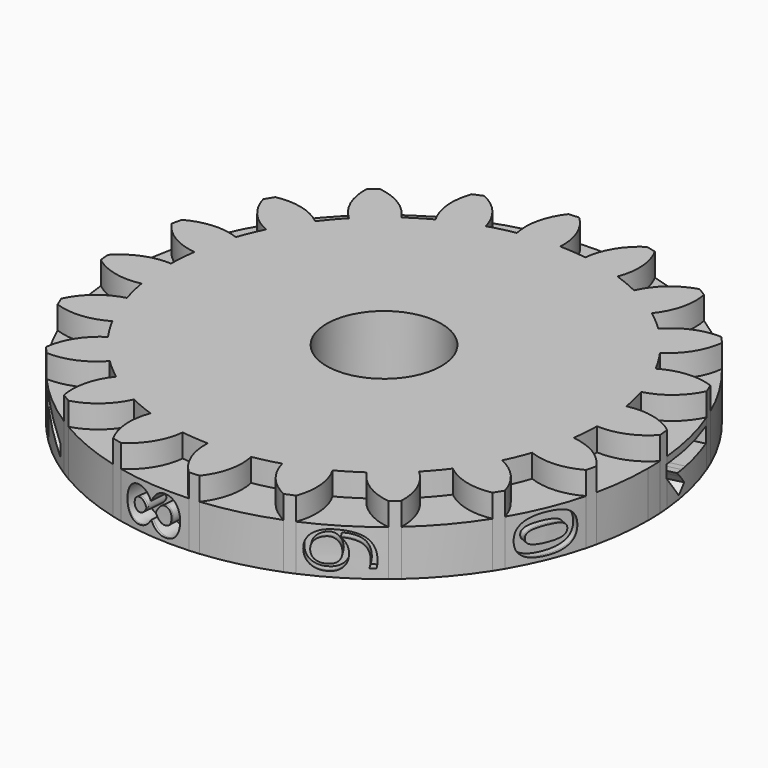
from build123d import *

# Parameters (mm, degrees)
F1_R          = 3.5
F1_R_2        = 2.5
F2_DEPTH      = 3
F3_DEPTH      = 2
F4_DEPTH      = 1
F8_TEXT_SIZE  = 3.422459893
F9_DEPTH      = 0.25
F11_TEXT_SIZE = 3.242330425
F12_DEPTH     = 0.25
F14_TEXT_SIZE = 3.3822665884
F15_DEPTH     = 0.25
F17_TEXT_SIZE = 3.3391304348
F18_DEPTH     = 0.25
F20_TEXT_SIZE = 4.3570347958
F21_DEPTH     = 0.9
F23_TEXT_SIZE = 3.3635036496
F24_DEPTH     = 0.25
F26_TEXT_SIZE = 3.4740651387
F27_DEPTH     = 0.25
F29_TEXT_SIZE = 3.3576216846
F30_DEPTH     = 0.9
F32_TEXT_SIZE = 3.3391304348
F33_DEPTH     = 0.25
F35_TEXT_SIZE = 3.3391304348
F36_DEPTH     = 0.25
F37_R         = 3.5
F37_R_2       = 2.5
F38_DEPTH     = 1


# Not quite as in the source:
# - Text() gives the source's letters only with a copy of the font that has no kerning and outlines rounded to 1/6400 em; it was checked with that copy


with BuildPart() as f2:
    # F1 (on Top) → F2 (new body)
    with BuildSketch(Plane.XY):
        with BuildLine():
            ThreePointArc((9.4078443957, -0.1531520845), (9.4087792756, -0.0765785786), (9.4090909091, 0))
            ThreePointArc((9.4090909091, 0), (9.3737668631, 0.8145468262), (9.2680599554, 1.6229776334))
            ThreePointArc((9.2680599554, 1.6229776334), (9.1491169783, 2.1965086508), (8.9947183137, 2.7615275108))
            ThreePointArc((8.9947183137, 2.7615275108), (8.6928665104, 3.6007032045), (8.3129211438, 4.4075314852))
            ThreePointArc((8.3129211438, 4.4075314852), (8.0225688191, 4.9162364953), (7.7011265332, 5.4058895526))
            ThreePointArc((7.7011265332, 5.4058895526), (7.1547288581, 6.1107157275), (6.5440556911, 6.7606454461))
            ThreePointArc((6.5440556911, 6.7606454461), (6.1107157275, 7.1547288581), (5.6536948308, 7.52108546))
            ThreePointArc((5.6536948308, 7.52108546), (4.9162364953, 8.0225688191), (4.1346124722, 8.4519803265))
            ThreePointArc((4.1346124722, 8.4519803265), (3.6007032045, 8.6928665104), (3.0528400867, 8.90006512))
            ThreePointArc((3.0528400867, 8.90006512), (2.1965086508, 9.1491169783), (1.320444577, 9.3159764842))
            ThreePointArc((1.320444577, 9.3159764842), (0.7382287643, 9.3800858219), (0.1531520845, 9.4078443957))
            ThreePointArc((0.1531520845, 9.4078443957), (-0.7382287643, 9.3800858219), (-1.6229776334, 9.2680599554))
            ThreePointArc((-1.6229776334, 9.2680599554), (-2.1965086508, 9.1491169783), (-2.7615275108, 8.9947183137))
            ThreePointArc((-2.7615275108, 8.9947183137), (-3.6007032045, 8.6928665104), (-4.4075314852, 8.3129211438))
            ThreePointArc((-4.4075314852, 8.3129211438), (-4.9162364953, 8.0225688191), (-5.4058895526, 7.7011265332))
            ThreePointArc((-5.4058895526, 7.7011265332), (-6.1107157275, 7.1547288581), (-6.7606454461, 6.5440556911))
            ThreePointArc((-6.7606454461, 6.5440556911), (-7.1547288581, 6.1107157275), (-7.52108546, 5.6536948308))
            ThreePointArc((-7.52108546, 5.6536948308), (-8.0225688191, 4.9162364953), (-8.4519803265, 4.1346124722))
            ThreePointArc((-8.4519803265, 4.1346124722), (-8.6928665104, 3.6007032045), (-8.90006512, 3.0528400867))
            ThreePointArc((-8.90006512, 3.0528400867), (-9.1491169783, 2.1965086508), (-9.3159764842, 1.320444577))
            ThreePointArc((-9.3159764842, 1.320444577), (-9.3800858219, 0.7382287643), (-9.4078443957, 0.1531520845))
            ThreePointArc((-9.4078443957, 0.1531520845), (-9.3800858219, -0.7382287643), (-9.2680599554, -1.6229776334))
            ThreePointArc((-9.2680599554, -1.6229776334), (-9.1491169783, -2.1965086508), (-8.9947183137, -2.7615275108))
            ThreePointArc((-8.9947183137, -2.7615275108), (-8.6928665104, -3.6007032045), (-8.3129211438, -4.4075314852))
            ThreePointArc((-8.3129211438, -4.4075314852), (-8.0225688191, -4.9162364953), (-7.7011265332, -5.4058895526))
            ThreePointArc((-7.7011265332, -5.4058895526), (-7.1547288581, -6.1107157275), (-6.5440556911, -6.7606454461))
            ThreePointArc((-6.5440556911, -6.7606454461), (-6.1107157275, -7.1547288581), (-5.6536948308, -7.52108546))
            ThreePointArc((-5.6536948308, -7.52108546), (-4.9162364953, -8.0225688191), (-4.1346124722, -8.4519803265))
            ThreePointArc((-4.1346124722, -8.4519803265), (-3.6007032045, -8.6928665104), (-3.0528400867, -8.90006512))
            ThreePointArc((-3.0528400867, -8.90006512), (-2.1965086508, -9.1491169783), (-1.320444577, -9.3159764842))
            ThreePointArc((-1.320444577, -9.3159764842), (-0.7382287643, -9.3800858219), (-0.1531520845, -9.4078443957))
            ThreePointArc((-0.1531520845, -9.4078443957), (0.7382287643, -9.3800858219), (1.6229776334, -9.2680599554))
            ThreePointArc((1.6229776334, -9.2680599554), (2.1965086508, -9.1491169783), (2.7615275108, -8.9947183137))
            ThreePointArc((2.7615275108, -8.9947183137), (3.6007032045, -8.6928665104), (4.4075314852, -8.3129211438))
            ThreePointArc((4.4075314852, -8.3129211438), (4.9162364953, -8.0225688191), (5.4058895526, -7.7011265332))
            ThreePointArc((5.4058895526, -7.7011265332), (6.1107157275, -7.1547288581), (6.7606454461, -6.5440556911))
            ThreePointArc((6.7606454461, -6.5440556911), (7.1547288581, -6.1107157275), (7.52108546, -5.6536948308))
            ThreePointArc((7.52108546, -5.6536948308), (8.0225688191, -4.9162364953), (8.4519803265, -4.1346124722))
            ThreePointArc((8.4519803265, -4.1346124722), (8.6928665104, -3.6007032045), (8.90006512, -3.0528400867))
            ThreePointArc((8.90006512, -3.0528400867), (9.1491169783, -2.1965086508), (9.3159764842, -1.320444577))
            ThreePointArc((9.3159764842, -1.320444577), (9.3800858219, -0.7382287643), (9.4078443957, -0.1531520845))
        make_face()
        Circle(F1_R, mode=Mode.SUBTRACT)
        Circle(F1_R)
        Circle(F1_R_2, mode=Mode.SUBTRACT)
        with BuildLine():
            ThreePointArc((-9.2680599554, -1.6229776334), (-9.3800858219, -0.7382287643), (-9.4078443957, 0.1531520845))
            ThreePointArc((-9.4078443957, 0.1531520845), (-10.5374998224, -0.0317997207), (-11.4797736507, -0.6817601701))
            Line((-11.4797736507, -0.6817601701), (-11.4450893749, -1.1224656787))
            ThreePointArc((-11.4450893749, -1.1224656787), (-10.4127402859, -1.6170199342), (-9.2680599554, -1.6229776334))
        make_face()
        with BuildLine():
            ThreePointArc((-9.3159764842, 1.320444577), (-9.1491169783, 2.1965086508), (-8.90006512, 3.0528400867))
            ThreePointArc((-8.90006512, 3.0528400867), (-10.0315845257, 3.2260231917), (-11.1285890147, 2.8990526973))
            Line((-11.1285890147, 2.8990526973), (-11.2317877999, 2.469198821))
            ThreePointArc((-11.2317877999, 2.469198821), (-10.4027911413, 1.679836361), (-9.3159764842, 1.320444577))
        make_face()
    extrude(amount=-F2_DEPTH)

    # F1 (on Top) → F3 (join)
    with BuildSketch(Plane.XY):
        with BuildLine():
            ThreePointArc((9.4078443957, -0.1531520845), (9.4087792756, -0.0765785786), (9.4090909091, 0))
            ThreePointArc((9.4090909091, 0), (9.3737668631, 0.8145468262), (9.2680599554, 1.6229776334))
            ThreePointArc((9.2680599554, 1.6229776334), (9.1491169783, 2.1965086508), (8.9947183137, 2.7615275108))
            ThreePointArc((8.9947183137, 2.7615275108), (8.6928665104, 3.6007032045), (8.3129211438, 4.4075314852))
            ThreePointArc((8.3129211438, 4.4075314852), (8.0225688191, 4.9162364953), (7.7011265332, 5.4058895526))
            ThreePointArc((7.7011265332, 5.4058895526), (7.1547288581, 6.1107157275), (6.5440556911, 6.7606454461))
            ThreePointArc((6.5440556911, 6.7606454461), (6.1107157275, 7.1547288581), (5.6536948308, 7.52108546))
            ThreePointArc((5.6536948308, 7.52108546), (4.9162364953, 8.0225688191), (4.1346124722, 8.4519803265))
            ThreePointArc((4.1346124722, 8.4519803265), (3.6007032045, 8.6928665104), (3.0528400867, 8.90006512))
            ThreePointArc((3.0528400867, 8.90006512), (2.1965086508, 9.1491169783), (1.320444577, 9.3159764842))
            ThreePointArc((1.320444577, 9.3159764842), (0.7382287643, 9.3800858219), (0.1531520845, 9.4078443957))
            ThreePointArc((0.1531520845, 9.4078443957), (-0.7382287643, 9.3800858219), (-1.6229776334, 9.2680599554))
            ThreePointArc((-1.6229776334, 9.2680599554), (-2.1965086508, 9.1491169783), (-2.7615275108, 8.9947183137))
            ThreePointArc((-2.7615275108, 8.9947183137), (-3.6007032045, 8.6928665104), (-4.4075314852, 8.3129211438))
            ThreePointArc((-4.4075314852, 8.3129211438), (-4.9162364953, 8.0225688191), (-5.4058895526, 7.7011265332))
            ThreePointArc((-5.4058895526, 7.7011265332), (-6.1107157275, 7.1547288581), (-6.7606454461, 6.5440556911))
            ThreePointArc((-6.7606454461, 6.5440556911), (-7.1547288581, 6.1107157275), (-7.52108546, 5.6536948308))
            ThreePointArc((-7.52108546, 5.6536948308), (-8.0225688191, 4.9162364953), (-8.4519803265, 4.1346124722))
            ThreePointArc((-8.4519803265, 4.1346124722), (-8.6928665104, 3.6007032045), (-8.90006512, 3.0528400867))
            ThreePointArc((-8.90006512, 3.0528400867), (-9.1491169783, 2.1965086508), (-9.3159764842, 1.320444577))
            ThreePointArc((-9.3159764842, 1.320444577), (-9.3800858219, 0.7382287643), (-9.4078443957, 0.1531520845))
            ThreePointArc((-9.4078443957, 0.1531520845), (-9.3800858219, -0.7382287643), (-9.2680599554, -1.6229776334))
            ThreePointArc((-9.2680599554, -1.6229776334), (-9.1491169783, -2.1965086508), (-8.9947183137, -2.7615275108))
            ThreePointArc((-8.9947183137, -2.7615275108), (-8.6928665104, -3.6007032045), (-8.3129211438, -4.4075314852))
            ThreePointArc((-8.3129211438, -4.4075314852), (-8.0225688191, -4.9162364953), (-7.7011265332, -5.4058895526))
            ThreePointArc((-7.7011265332, -5.4058895526), (-7.1547288581, -6.1107157275), (-6.5440556911, -6.7606454461))
            ThreePointArc((-6.5440556911, -6.7606454461), (-6.1107157275, -7.1547288581), (-5.6536948308, -7.52108546))
            ThreePointArc((-5.6536948308, -7.52108546), (-4.9162364953, -8.0225688191), (-4.1346124722, -8.4519803265))
            ThreePointArc((-4.1346124722, -8.4519803265), (-3.6007032045, -8.6928665104), (-3.0528400867, -8.90006512))
            ThreePointArc((-3.0528400867, -8.90006512), (-2.1965086508, -9.1491169783), (-1.320444577, -9.3159764842))
            ThreePointArc((-1.320444577, -9.3159764842), (-0.7382287643, -9.3800858219), (-0.1531520845, -9.4078443957))
            ThreePointArc((-0.1531520845, -9.4078443957), (0.7382287643, -9.3800858219), (1.6229776334, -9.2680599554))
            ThreePointArc((1.6229776334, -9.2680599554), (2.1965086508, -9.1491169783), (2.7615275108, -8.9947183137))
            ThreePointArc((2.7615275108, -8.9947183137), (3.6007032045, -8.6928665104), (4.4075314852, -8.3129211438))
            ThreePointArc((4.4075314852, -8.3129211438), (4.9162364953, -8.0225688191), (5.4058895526, -7.7011265332))
            ThreePointArc((5.4058895526, -7.7011265332), (6.1107157275, -7.1547288581), (6.7606454461, -6.5440556911))
            ThreePointArc((6.7606454461, -6.5440556911), (7.1547288581, -6.1107157275), (7.52108546, -5.6536948308))
            ThreePointArc((7.52108546, -5.6536948308), (8.0225688191, -4.9162364953), (8.4519803265, -4.1346124722))
            ThreePointArc((8.4519803265, -4.1346124722), (8.6928665104, -3.6007032045), (8.90006512, -3.0528400867))
            ThreePointArc((8.90006512, -3.0528400867), (9.1491169783, -2.1965086508), (9.3159764842, -1.320444577))
            ThreePointArc((9.3159764842, -1.320444577), (9.3800858219, -0.7382287643), (9.4078443957, -0.1531520845))
        make_face()
        Circle(F1_R, mode=Mode.SUBTRACT)
        Circle(F1_R)
        Circle(F1_R_2, mode=Mode.SUBTRACT)
        with BuildLine():
            ThreePointArc((4.195837602, -10.7072380574), (3.286509855, -10.0119312174), (2.7615275108, -8.9947183137))
            ThreePointArc((2.7615275108, -8.9947183137), (2.1965086508, -9.1491169783), (1.6229776334, -9.2680599554))
            ThreePointArc((1.6229776334, -9.2680599554), (1.6170199342, -10.4127402859), (1.1224656787, -11.4450893749))
            ThreePointArc((1.1224656787, -11.4450893749), (2.6846216843, -11.1822540846), (4.195837602, -10.7072380574))
        make_face()
        with BuildLine():
            ThreePointArc((7.2991972152, -8.8866034014), (6.2195135061, -8.5063250277), (5.4058895526, -7.7011265332))
            ThreePointArc((5.4058895526, -7.7011265332), (4.9162364953, -8.0225688191), (4.4075314852, -8.3129211438))
            ThreePointArc((4.4075314852, -8.3129211438), (4.7555910517, -9.4034178615), (4.604255417, -10.5380658593))
            ThreePointArc((4.604255417, -10.5380658593), (6.0087334942, -9.8053618901), (7.2991972152, -8.8866034014))
        make_face()
        with BuildLine():
            ThreePointArc((9.6880605486, -6.1960860878), (8.5437078414, -6.1680604771), (7.52108546, -5.6536948308))
            ThreePointArc((7.52108546, -5.6536948308), (7.1547288581, -6.1107157275), (6.7606454461, -6.5440556911))
            ThreePointArc((6.7606454461, -6.5440556911), (7.428651783, -7.4736233793), (7.6353485554, -8.5995030343))
            ThreePointArc((7.6353485554, -8.5995030343), (8.7446686044, -7.4686525558), (9.6880605486, -6.1960860878))
        make_face()
        with BuildLine():
            ThreePointArc((11.1285890147, -2.8990526973), (10.0315845257, -3.2260231917), (8.90006512, -3.0528400867))
            ThreePointArc((8.90006512, -3.0528400867), (8.6928665104, -3.6007032045), (8.4519803265, -4.1346124722))
            ThreePointArc((8.4519803265, -4.1346124722), (9.3745443193, -4.812258569), (9.9190405786, -5.8191609361))
            ThreePointArc((9.9190405786, -5.8191609361), (10.6246146239, -4.4008594722), (11.1285890147, -2.8990526973))
        make_face()
        with BuildLine():
            ThreePointArc((11.4797736507, 0.6817601701), (10.5374998224, 0.0317997207), (9.4078443957, -0.1531520845))
            ThreePointArc((9.4078443957, -0.1531520845), (9.3800858219, -0.7382287643), (9.3159764842, -1.320444577))
            ThreePointArc((9.3159764842, -1.320444577), (10.4027911413, -1.679836361), (11.2317877999, -2.469198821))
            ThreePointArc((11.2317877999, -2.469198821), (11.4327503187, -1.2418615665), (11.5, 0))
            ThreePointArc((11.5, 0), (11.4949423005, 0.3410300701), (11.4797736507, 0.6817601701))
        make_face()
        with BuildLine():
            ThreePointArc((8.9947183137, 2.7615275108), (9.1491169783, 2.1965086508), (9.2680599554, 1.6229776334))
            ThreePointArc((9.2680599554, 1.6229776334), (10.4127402859, 1.6170199342), (11.4450893749, 1.1224656787))
            ThreePointArc((11.4450893749, 1.1224656787), (11.1822540846, 2.6846216843), (10.7072380574, 4.195837602))
            ThreePointArc((10.7072380574, 4.195837602), (10.0119312174, 3.286509855), (8.9947183137, 2.7615275108))
        make_face()
        with BuildLine():
            ThreePointArc((7.7011265332, 5.4058895526), (8.0225688191, 4.9162364953), (8.3129211438, 4.4075314852))
            ThreePointArc((8.3129211438, 4.4075314852), (9.4034178615, 4.7555910517), (10.5380658593, 4.604255417))
            ThreePointArc((10.5380658593, 4.604255417), (9.8053618901, 6.0087334942), (8.8866034014, 7.2991972152))
            ThreePointArc((8.8866034014, 7.2991972152), (8.5063250277, 6.2195135061), (7.7011265332, 5.4058895526))
        make_face()
        with BuildLine():
            ThreePointArc((5.6536948308, 7.52108546), (6.1107157275, 7.1547288581), (6.5440556911, 6.7606454461))
            ThreePointArc((6.5440556911, 6.7606454461), (7.4736233793, 7.428651783), (8.5995030343, 7.6353485554))
            ThreePointArc((8.5995030343, 7.6353485554), (7.4686525558, 8.7446686044), (6.1960860878, 9.6880605486))
            ThreePointArc((6.1960860878, 9.6880605486), (6.1680604771, 8.5437078414), (5.6536948308, 7.52108546))
        make_face()
        with BuildLine():
            ThreePointArc((3.0528400867, 8.90006512), (3.6007032045, 8.6928665104), (4.1346124722, 8.4519803265))
            ThreePointArc((4.1346124722, 8.4519803265), (4.812258569, 9.3745443193), (5.8191609361, 9.9190405786))
            ThreePointArc((5.8191609361, 9.9190405786), (4.4008594722, 10.6246146239), (2.8990526973, 11.1285890147))
            ThreePointArc((2.8990526973, 11.1285890147), (3.2260231917, 10.0315845257), (3.0528400867, 8.90006512))
        make_face()
        with BuildLine():
            ThreePointArc((0.1531520845, 9.4078443957), (0.7382287643, 9.3800858219), (1.320444577, 9.3159764842))
            ThreePointArc((1.320444577, 9.3159764842), (1.679836361, 10.4027911413), (2.469198821, 11.2317877999))
            ThreePointArc((2.469198821, 11.2317877999), (0.9022796009, 11.4645493379), (-0.6817601701, 11.4797736507))
            ThreePointArc((-0.6817601701, 11.4797736507), (-0.0317997207, 10.5374998224), (0.1531520845, 9.4078443957))
        make_face()
        with BuildLine():
            ThreePointArc((-2.7615275108, 8.9947183137), (-2.1965086508, 9.1491169783), (-1.6229776334, 9.2680599554))
            ThreePointArc((-1.6229776334, 9.2680599554), (-1.6170199342, 10.4127402859), (-1.1224656787, 11.4450893749))
            ThreePointArc((-1.1224656787, 11.4450893749), (-2.6846216843, 11.1822540846), (-4.195837602, 10.7072380574))
            ThreePointArc((-4.195837602, 10.7072380574), (-3.286509855, 10.0119312174), (-2.7615275108, 8.9947183137))
        make_face()
        with BuildLine():
            ThreePointArc((-5.4058895526, 7.7011265332), (-4.9162364953, 8.0225688191), (-4.4075314852, 8.3129211438))
            ThreePointArc((-4.4075314852, 8.3129211438), (-4.7555910517, 9.4034178615), (-4.604255417, 10.5380658593))
            ThreePointArc((-4.604255417, 10.5380658593), (-4.7705084102, 10.4638544289), (-4.935565714, 10.3870203178))
            ThreePointArc((-4.935565714, 10.3870203178), (-6.1632109094, 9.7090077395), (-7.2991972152, 8.8866034014))
            ThreePointArc((-7.2991972152, 8.8866034014), (-6.2195135061, 8.5063250277), (-5.4058895526, 7.7011265332))
        make_face()
        with BuildLine():
            ThreePointArc((-7.52108546, 5.6536948308), (-7.1547288581, 6.1107157275), (-6.7606454461, 6.5440556911))
            ThreePointArc((-6.7606454461, 6.5440556911), (-7.428651783, 7.4736233793), (-7.6353485554, 8.5995030343))
            ThreePointArc((-7.6353485554, 8.5995030343), (-8.7446686044, 7.4686525558), (-9.6880605486, 6.1960860878))
            ThreePointArc((-9.6880605486, 6.1960860878), (-8.5437078414, 6.1680604771), (-7.52108546, 5.6536948308))
        make_face()
        with BuildLine():
            ThreePointArc((-8.90006512, 3.0528400867), (-8.6928665104, 3.6007032045), (-8.4519803265, 4.1346124722))
            ThreePointArc((-8.4519803265, 4.1346124722), (-9.3745443193, 4.812258569), (-9.9190405786, 5.8191609361))
            ThreePointArc((-9.9190405786, 5.8191609361), (-10.6246146239, 4.4008594722), (-11.1285890147, 2.8990526973))
            ThreePointArc((-11.1285890147, 2.8990526973), (-10.0315845257, 3.2260231917), (-8.90006512, 3.0528400867))
        make_face()
        with BuildLine():
            ThreePointArc((-9.4078443957, 0.1531520845), (-9.3800858219, 0.7382287643), (-9.3159764842, 1.320444577))
            ThreePointArc((-9.3159764842, 1.320444577), (-10.4027911413, 1.679836361), (-11.2317877999, 2.469198821))
            ThreePointArc((-11.2317877999, 2.469198821), (-11.4645493379, 0.9022796009), (-11.4797736507, -0.6817601701))
            ThreePointArc((-11.4797736507, -0.6817601701), (-10.5374998224, -0.0317997207), (-9.4078443957, 0.1531520845))
        make_face()
        with BuildLine():
            ThreePointArc((-10.7072380574, -4.195837602), (-10.0119312174, -3.286509855), (-8.9947183137, -2.7615275108))
            ThreePointArc((-8.9947183137, -2.7615275108), (-9.1491169783, -2.1965086508), (-9.2680599554, -1.6229776334))
            ThreePointArc((-9.2680599554, -1.6229776334), (-10.4127402859, -1.6170199342), (-11.4450893749, -1.1224656787))
            ThreePointArc((-11.4450893749, -1.1224656787), (-11.1822540846, -2.6846216843), (-10.7072380574, -4.195837602))
        make_face()
        with BuildLine():
            ThreePointArc((-8.8866034014, -7.2991972152), (-8.5063250277, -6.2195135061), (-7.7011265332, -5.4058895526))
            ThreePointArc((-7.7011265332, -5.4058895526), (-8.0225688191, -4.9162364953), (-8.3129211438, -4.4075314852))
            ThreePointArc((-8.3129211438, -4.4075314852), (-9.4034178615, -4.7555910517), (-10.5380658593, -4.604255417))
            ThreePointArc((-10.5380658593, -4.604255417), (-9.8053618901, -6.0087334942), (-8.8866034014, -7.2991972152))
        make_face()
        with BuildLine():
            ThreePointArc((-6.1960860878, -9.6880605486), (-6.1680604771, -8.5437078414), (-5.6536948308, -7.52108546))
            ThreePointArc((-5.6536948308, -7.52108546), (-6.1107157275, -7.1547288581), (-6.5440556911, -6.7606454461))
            ThreePointArc((-6.5440556911, -6.7606454461), (-7.4736233793, -7.428651783), (-8.5995030343, -7.6353485554))
            ThreePointArc((-8.5995030343, -7.6353485554), (-7.4686525558, -8.7446686044), (-6.1960860878, -9.6880605486))
        make_face()
        with BuildLine():
            ThreePointArc((-2.8990526973, -11.1285890147), (-3.2260231917, -10.0315845257), (-3.0528400867, -8.90006512))
            ThreePointArc((-3.0528400867, -8.90006512), (-3.6007032045, -8.6928665104), (-4.1346124722, -8.4519803265))
            ThreePointArc((-4.1346124722, -8.4519803265), (-4.812258569, -9.3745443193), (-5.8191609361, -9.9190405786))
            ThreePointArc((-5.8191609361, -9.9190405786), (-4.4008594722, -10.6246146239), (-2.8990526973, -11.1285890147))
        make_face()
        with BuildLine():
            ThreePointArc((0.6817601701, -11.4797736507), (0.0317997207, -10.5374998224), (-0.1531520845, -9.4078443957))
            ThreePointArc((-0.1531520845, -9.4078443957), (-0.7382287643, -9.3800858219), (-1.320444577, -9.3159764842))
            ThreePointArc((-1.320444577, -9.3159764842), (-1.679836361, -10.4027911413), (-2.469198821, -11.2317877999))
            ThreePointArc((-2.469198821, -11.2317877999), (-0.9022796009, -11.4645493379), (0.6817601701, -11.4797736507))
        make_face()
        with BuildLine():
            ThreePointArc((4.604255417, -10.5380658593), (4.7555910517, -9.4034178615), (4.4075314852, -8.3129211438))
            ThreePointArc((4.4075314852, -8.3129211438), (3.6007032045, -8.6928665104), (2.7615275108, -8.9947183137))
            ThreePointArc((2.7615275108, -8.9947183137), (3.286509855, -10.0119312174), (4.195837602, -10.7072380574))
            Line((4.195837602, -10.7072380574), (4.604255417, -10.5380658593))
        make_face()
        with BuildLine():
            ThreePointArc((7.6353485554, -8.5995030343), (7.428651783, -7.4736233793), (6.7606454461, -6.5440556911))
            ThreePointArc((6.7606454461, -6.5440556911), (6.1107157275, -7.1547288581), (5.4058895526, -7.7011265332))
            ThreePointArc((5.4058895526, -7.7011265332), (6.2195135061, -8.5063250277), (7.2991972152, -8.8866034014))
            Line((7.2991972152, -8.8866034014), (7.6353485554, -8.5995030343))
        make_face()
        with BuildLine():
            ThreePointArc((9.9190405786, -5.8191609361), (9.3745443193, -4.812258569), (8.4519803265, -4.1346124722))
            ThreePointArc((8.4519803265, -4.1346124722), (8.0225688191, -4.9162364953), (7.52108546, -5.6536948308))
            ThreePointArc((7.52108546, -5.6536948308), (8.5437078414, -6.1680604771), (9.6880605486, -6.1960860878))
            Line((9.6880605486, -6.1960860878), (9.9190405786, -5.8191609361))
        make_face()
        with BuildLine():
            ThreePointArc((11.2317877999, -2.469198821), (10.4027911413, -1.679836361), (9.3159764842, -1.320444577))
            ThreePointArc((9.3159764842, -1.320444577), (9.1491169783, -2.1965086508), (8.90006512, -3.0528400867))
            ThreePointArc((8.90006512, -3.0528400867), (10.0315845257, -3.2260231917), (11.1285890147, -2.8990526973))
            Line((11.1285890147, -2.8990526973), (11.2317877999, -2.469198821))
        make_face()
        with BuildLine():
            ThreePointArc((9.2680599554, 1.6229776334), (9.3737668631, 0.8145468262), (9.4090909091, 0))
            ThreePointArc((9.4090909091, 0), (9.4087792756, -0.0765785786), (9.4078443957, -0.1531520845))
            ThreePointArc((9.4078443957, -0.1531520845), (10.5374998224, 0.0317997207), (11.4797736507, 0.6817601701))
            Line((11.4797736507, 0.6817601701), (11.4450893749, 1.1224656787))
            ThreePointArc((11.4450893749, 1.1224656787), (10.4127402859, 1.6170199342), (9.2680599554, 1.6229776334))
        make_face()
        with BuildLine():
            ThreePointArc((8.3129211438, 4.4075314852), (8.6928665104, 3.6007032045), (8.9947183137, 2.7615275108))
            ThreePointArc((8.9947183137, 2.7615275108), (10.0119312174, 3.286509855), (10.7072380574, 4.195837602))
            Line((10.7072380574, 4.195837602), (10.5380658593, 4.604255417))
            ThreePointArc((10.5380658593, 4.604255417), (9.4034178615, 4.7555910517), (8.3129211438, 4.4075314852))
        make_face()
        with BuildLine():
            ThreePointArc((6.5440556911, 6.7606454461), (7.1547288581, 6.1107157275), (7.7011265332, 5.4058895526))
            ThreePointArc((7.7011265332, 5.4058895526), (8.5063250277, 6.2195135061), (8.8866034014, 7.2991972152))
            Line((8.8866034014, 7.2991972152), (8.5995030343, 7.6353485554))
            ThreePointArc((8.5995030343, 7.6353485554), (7.4736233793, 7.428651783), (6.5440556911, 6.7606454461))
        make_face()
        with BuildLine():
            ThreePointArc((4.1346124722, 8.4519803265), (4.9162364953, 8.0225688191), (5.6536948308, 7.52108546))
            ThreePointArc((5.6536948308, 7.52108546), (6.1680604771, 8.5437078414), (6.1960860878, 9.6880605486))
            Line((6.1960860878, 9.6880605486), (5.8191609361, 9.9190405786))
            ThreePointArc((5.8191609361, 9.9190405786), (4.812258569, 9.3745443193), (4.1346124722, 8.4519803265))
        make_face()
        with BuildLine():
            ThreePointArc((1.320444577, 9.3159764842), (2.1965086508, 9.1491169783), (3.0528400867, 8.90006512))
            ThreePointArc((3.0528400867, 8.90006512), (3.2260231917, 10.0315845257), (2.8990526973, 11.1285890147))
            Line((2.8990526973, 11.1285890147), (2.469198821, 11.2317877999))
            ThreePointArc((2.469198821, 11.2317877999), (1.679836361, 10.4027911413), (1.320444577, 9.3159764842))
        make_face()
        with BuildLine():
            ThreePointArc((-1.6229776334, 9.2680599554), (-0.7382287643, 9.3800858219), (0.1531520845, 9.4078443957))
            ThreePointArc((0.1531520845, 9.4078443957), (-0.0317997207, 10.5374998224), (-0.6817601701, 11.4797736507))
            Line((-0.6817601701, 11.4797736507), (-1.1224656787, 11.4450893749))
            ThreePointArc((-1.1224656787, 11.4450893749), (-1.6170199342, 10.4127402859), (-1.6229776334, 9.2680599554))
        make_face()
        with BuildLine():
            ThreePointArc((-4.4075314852, 8.3129211438), (-3.6007032045, 8.6928665104), (-2.7615275108, 8.9947183137))
            ThreePointArc((-2.7615275108, 8.9947183137), (-3.286509855, 10.0119312174), (-4.195837602, 10.7072380574))
            Line((-4.195837602, 10.7072380574), (-4.604255417, 10.5380658593))
            ThreePointArc((-4.604255417, 10.5380658593), (-4.7555910517, 9.4034178615), (-4.4075314852, 8.3129211438))
        make_face()
        with BuildLine():
            ThreePointArc((-6.7606454461, 6.5440556911), (-6.1107157275, 7.1547288581), (-5.4058895526, 7.7011265332))
            ThreePointArc((-5.4058895526, 7.7011265332), (-6.2195135061, 8.5063250277), (-7.2991972152, 8.8866034014))
            Line((-7.2991972152, 8.8866034014), (-7.6353485554, 8.5995030343))
            ThreePointArc((-7.6353485554, 8.5995030343), (-7.428651783, 7.4736233793), (-6.7606454461, 6.5440556911))
        make_face()
        with BuildLine():
            ThreePointArc((-8.4519803265, 4.1346124722), (-8.0225688191, 4.9162364953), (-7.52108546, 5.6536948308))
            ThreePointArc((-7.52108546, 5.6536948308), (-8.5437078414, 6.1680604771), (-9.6880605486, 6.1960860878))
            Line((-9.6880605486, 6.1960860878), (-9.9190405786, 5.8191609361))
            ThreePointArc((-9.9190405786, 5.8191609361), (-9.3745443193, 4.812258569), (-8.4519803265, 4.1346124722))
        make_face()
        with BuildLine():
            ThreePointArc((-9.3159764842, 1.320444577), (-9.1491169783, 2.1965086508), (-8.90006512, 3.0528400867))
            ThreePointArc((-8.90006512, 3.0528400867), (-10.0315845257, 3.2260231917), (-11.1285890147, 2.8990526973))
            Line((-11.1285890147, 2.8990526973), (-11.2317877999, 2.469198821))
            ThreePointArc((-11.2317877999, 2.469198821), (-10.4027911413, 1.679836361), (-9.3159764842, 1.320444577))
        make_face()
        with BuildLine():
            ThreePointArc((-9.2680599554, -1.6229776334), (-9.3800858219, -0.7382287643), (-9.4078443957, 0.1531520845))
            ThreePointArc((-9.4078443957, 0.1531520845), (-10.5374998224, -0.0317997207), (-11.4797736507, -0.6817601701))
            Line((-11.4797736507, -0.6817601701), (-11.4450893749, -1.1224656787))
            ThreePointArc((-11.4450893749, -1.1224656787), (-10.4127402859, -1.6170199342), (-9.2680599554, -1.6229776334))
        make_face()
        with BuildLine():
            ThreePointArc((-10.5380658593, -4.604255417), (-9.4034178615, -4.7555910517), (-8.3129211438, -4.4075314852))
            ThreePointArc((-8.3129211438, -4.4075314852), (-8.6928665104, -3.6007032045), (-8.9947183137, -2.7615275108))
            ThreePointArc((-8.9947183137, -2.7615275108), (-10.0119312174, -3.286509855), (-10.7072380574, -4.195837602))
            Line((-10.7072380574, -4.195837602), (-10.5380658593, -4.604255417))
        make_face()
        with BuildLine():
            ThreePointArc((-8.5995030343, -7.6353485554), (-7.4736233793, -7.428651783), (-6.5440556911, -6.7606454461))
            ThreePointArc((-6.5440556911, -6.7606454461), (-7.1547288581, -6.1107157275), (-7.7011265332, -5.4058895526))
            ThreePointArc((-7.7011265332, -5.4058895526), (-8.5063250277, -6.2195135061), (-8.8866034014, -7.2991972152))
            Line((-8.8866034014, -7.2991972152), (-8.5995030343, -7.6353485554))
        make_face()
        with BuildLine():
            ThreePointArc((-5.8191609361, -9.9190405786), (-4.812258569, -9.3745443193), (-4.1346124722, -8.4519803265))
            ThreePointArc((-4.1346124722, -8.4519803265), (-4.9162364953, -8.0225688191), (-5.6536948308, -7.52108546))
            ThreePointArc((-5.6536948308, -7.52108546), (-6.1680604771, -8.5437078414), (-6.1960860878, -9.6880605486))
            Line((-6.1960860878, -9.6880605486), (-5.8191609361, -9.9190405786))
        make_face()
        with BuildLine():
            ThreePointArc((-2.469198821, -11.2317877999), (-1.679836361, -10.4027911413), (-1.320444577, -9.3159764842))
            ThreePointArc((-1.320444577, -9.3159764842), (-2.1965086508, -9.1491169783), (-3.0528400867, -8.90006512))
            ThreePointArc((-3.0528400867, -8.90006512), (-3.2260231917, -10.0315845257), (-2.8990526973, -11.1285890147))
            Line((-2.8990526973, -11.1285890147), (-2.469198821, -11.2317877999))
        make_face()
        with BuildLine():
            ThreePointArc((1.1224656787, -11.4450893749), (1.6170199342, -10.4127402859), (1.6229776334, -9.2680599554))
            ThreePointArc((1.6229776334, -9.2680599554), (0.7382287643, -9.3800858219), (-0.1531520845, -9.4078443957))
            ThreePointArc((-0.1531520845, -9.4078443957), (0.0317997207, -10.5374998224), (0.6817601701, -11.4797736507))
            Line((0.6817601701, -11.4797736507), (1.1224656787, -11.4450893749))
        make_face()
    extrude(amount=-F3_DEPTH)

    # F1 (on Top) → F4 (join)
    with BuildSketch(Plane.XY):
        with BuildLine():
            ThreePointArc((-1.6229776334, 9.2680599554), (-0.7382287643, 9.3800858219), (0.1531520845, 9.4078443957))
            ThreePointArc((0.1531520845, 9.4078443957), (-0.0317997207, 10.5374998224), (-0.6817601701, 11.4797736507))
            Line((-0.6817601701, 11.4797736507), (-1.1224656787, 11.4450893749))
            ThreePointArc((-1.1224656787, 11.4450893749), (-1.6170199342, 10.4127402859), (-1.6229776334, 9.2680599554))
        make_face()
        with BuildLine():
            ThreePointArc((9.4078443957, -0.1531520845), (9.4087792756, -0.0765785786), (9.4090909091, 0))
            ThreePointArc((9.4090909091, 0), (9.3737668631, 0.8145468262), (9.2680599554, 1.6229776334))
            ThreePointArc((9.2680599554, 1.6229776334), (9.1491169783, 2.1965086508), (8.9947183137, 2.7615275108))
            ThreePointArc((8.9947183137, 2.7615275108), (8.6928665104, 3.6007032045), (8.3129211438, 4.4075314852))
            ThreePointArc((8.3129211438, 4.4075314852), (8.0225688191, 4.9162364953), (7.7011265332, 5.4058895526))
            ThreePointArc((7.7011265332, 5.4058895526), (7.1547288581, 6.1107157275), (6.5440556911, 6.7606454461))
            ThreePointArc((6.5440556911, 6.7606454461), (6.1107157275, 7.1547288581), (5.6536948308, 7.52108546))
            ThreePointArc((5.6536948308, 7.52108546), (4.9162364953, 8.0225688191), (4.1346124722, 8.4519803265))
            ThreePointArc((4.1346124722, 8.4519803265), (3.6007032045, 8.6928665104), (3.0528400867, 8.90006512))
            ThreePointArc((3.0528400867, 8.90006512), (2.1965086508, 9.1491169783), (1.320444577, 9.3159764842))
            ThreePointArc((1.320444577, 9.3159764842), (0.7382287643, 9.3800858219), (0.1531520845, 9.4078443957))
            ThreePointArc((0.1531520845, 9.4078443957), (-0.7382287643, 9.3800858219), (-1.6229776334, 9.2680599554))
            ThreePointArc((-1.6229776334, 9.2680599554), (-2.1965086508, 9.1491169783), (-2.7615275108, 8.9947183137))
            ThreePointArc((-2.7615275108, 8.9947183137), (-3.6007032045, 8.6928665104), (-4.4075314852, 8.3129211438))
            ThreePointArc((-4.4075314852, 8.3129211438), (-4.9162364953, 8.0225688191), (-5.4058895526, 7.7011265332))
            ThreePointArc((-5.4058895526, 7.7011265332), (-6.1107157275, 7.1547288581), (-6.7606454461, 6.5440556911))
            ThreePointArc((-6.7606454461, 6.5440556911), (-7.1547288581, 6.1107157275), (-7.52108546, 5.6536948308))
            ThreePointArc((-7.52108546, 5.6536948308), (-8.0225688191, 4.9162364953), (-8.4519803265, 4.1346124722))
            ThreePointArc((-8.4519803265, 4.1346124722), (-8.6928665104, 3.6007032045), (-8.90006512, 3.0528400867))
            ThreePointArc((-8.90006512, 3.0528400867), (-9.1491169783, 2.1965086508), (-9.3159764842, 1.320444577))
            ThreePointArc((-9.3159764842, 1.320444577), (-9.3800858219, 0.7382287643), (-9.4078443957, 0.1531520845))
            ThreePointArc((-9.4078443957, 0.1531520845), (-9.3800858219, -0.7382287643), (-9.2680599554, -1.6229776334))
            ThreePointArc((-9.2680599554, -1.6229776334), (-9.1491169783, -2.1965086508), (-8.9947183137, -2.7615275108))
            ThreePointArc((-8.9947183137, -2.7615275108), (-8.6928665104, -3.6007032045), (-8.3129211438, -4.4075314852))
            ThreePointArc((-8.3129211438, -4.4075314852), (-8.0225688191, -4.9162364953), (-7.7011265332, -5.4058895526))
            ThreePointArc((-7.7011265332, -5.4058895526), (-7.1547288581, -6.1107157275), (-6.5440556911, -6.7606454461))
            ThreePointArc((-6.5440556911, -6.7606454461), (-6.1107157275, -7.1547288581), (-5.6536948308, -7.52108546))
            ThreePointArc((-5.6536948308, -7.52108546), (-4.9162364953, -8.0225688191), (-4.1346124722, -8.4519803265))
            ThreePointArc((-4.1346124722, -8.4519803265), (-3.6007032045, -8.6928665104), (-3.0528400867, -8.90006512))
            ThreePointArc((-3.0528400867, -8.90006512), (-2.1965086508, -9.1491169783), (-1.320444577, -9.3159764842))
            ThreePointArc((-1.320444577, -9.3159764842), (-0.7382287643, -9.3800858219), (-0.1531520845, -9.4078443957))
            ThreePointArc((-0.1531520845, -9.4078443957), (0.7382287643, -9.3800858219), (1.6229776334, -9.2680599554))
            ThreePointArc((1.6229776334, -9.2680599554), (2.1965086508, -9.1491169783), (2.7615275108, -8.9947183137))
            ThreePointArc((2.7615275108, -8.9947183137), (3.6007032045, -8.6928665104), (4.4075314852, -8.3129211438))
            ThreePointArc((4.4075314852, -8.3129211438), (4.9162364953, -8.0225688191), (5.4058895526, -7.7011265332))
            ThreePointArc((5.4058895526, -7.7011265332), (6.1107157275, -7.1547288581), (6.7606454461, -6.5440556911))
            ThreePointArc((6.7606454461, -6.5440556911), (7.1547288581, -6.1107157275), (7.52108546, -5.6536948308))
            ThreePointArc((7.52108546, -5.6536948308), (8.0225688191, -4.9162364953), (8.4519803265, -4.1346124722))
            ThreePointArc((8.4519803265, -4.1346124722), (8.6928665104, -3.6007032045), (8.90006512, -3.0528400867))
            ThreePointArc((8.90006512, -3.0528400867), (9.1491169783, -2.1965086508), (9.3159764842, -1.320444577))
            ThreePointArc((9.3159764842, -1.320444577), (9.3800858219, -0.7382287643), (9.4078443957, -0.1531520845))
        make_face()
        Circle(F1_R, mode=Mode.SUBTRACT)
        with BuildLine():
            ThreePointArc((-4.4075314852, 8.3129211438), (-3.6007032045, 8.6928665104), (-2.7615275108, 8.9947183137))
            ThreePointArc((-2.7615275108, 8.9947183137), (-3.286509855, 10.0119312174), (-4.195837602, 10.7072380574))
            Line((-4.195837602, 10.7072380574), (-4.604255417, 10.5380658593))
            ThreePointArc((-4.604255417, 10.5380658593), (-4.7555910517, 9.4034178615), (-4.4075314852, 8.3129211438))
        make_face()
        with BuildLine():
            ThreePointArc((-6.7606454461, 6.5440556911), (-6.1107157275, 7.1547288581), (-5.4058895526, 7.7011265332))
            ThreePointArc((-5.4058895526, 7.7011265332), (-6.2195135061, 8.5063250277), (-7.2991972152, 8.8866034014))
            Line((-7.2991972152, 8.8866034014), (-7.6353485554, 8.5995030343))
            ThreePointArc((-7.6353485554, 8.5995030343), (-7.428651783, 7.4736233793), (-6.7606454461, 6.5440556911))
        make_face()
        with BuildLine():
            ThreePointArc((-8.4519803265, 4.1346124722), (-8.0225688191, 4.9162364953), (-7.52108546, 5.6536948308))
            ThreePointArc((-7.52108546, 5.6536948308), (-8.5437078414, 6.1680604771), (-9.6880605486, 6.1960860878))
            Line((-9.6880605486, 6.1960860878), (-9.9190405786, 5.8191609361))
            ThreePointArc((-9.9190405786, 5.8191609361), (-9.3745443193, 4.812258569), (-8.4519803265, 4.1346124722))
        make_face()
        with BuildLine():
            ThreePointArc((-9.3159764842, 1.320444577), (-9.1491169783, 2.1965086508), (-8.90006512, 3.0528400867))
            ThreePointArc((-8.90006512, 3.0528400867), (-10.0315845257, 3.2260231917), (-11.1285890147, 2.8990526973))
            Line((-11.1285890147, 2.8990526973), (-11.2317877999, 2.469198821))
            ThreePointArc((-11.2317877999, 2.469198821), (-10.4027911413, 1.679836361), (-9.3159764842, 1.320444577))
        make_face()
        with BuildLine():
            ThreePointArc((-9.2680599554, -1.6229776334), (-9.3800858219, -0.7382287643), (-9.4078443957, 0.1531520845))
            ThreePointArc((-9.4078443957, 0.1531520845), (-10.5374998224, -0.0317997207), (-11.4797736507, -0.6817601701))
            Line((-11.4797736507, -0.6817601701), (-11.4450893749, -1.1224656787))
            ThreePointArc((-11.4450893749, -1.1224656787), (-10.4127402859, -1.6170199342), (-9.2680599554, -1.6229776334))
        make_face()
        with BuildLine():
            ThreePointArc((-10.5380658593, -4.604255417), (-9.4034178615, -4.7555910517), (-8.3129211438, -4.4075314852))
            ThreePointArc((-8.3129211438, -4.4075314852), (-8.6928665104, -3.6007032045), (-8.9947183137, -2.7615275108))
            ThreePointArc((-8.9947183137, -2.7615275108), (-10.0119312174, -3.286509855), (-10.7072380574, -4.195837602))
            Line((-10.7072380574, -4.195837602), (-10.5380658593, -4.604255417))
        make_face()
        with BuildLine():
            ThreePointArc((-8.5995030343, -7.6353485554), (-7.4736233793, -7.428651783), (-6.5440556911, -6.7606454461))
            ThreePointArc((-6.5440556911, -6.7606454461), (-7.1547288581, -6.1107157275), (-7.7011265332, -5.4058895526))
            ThreePointArc((-7.7011265332, -5.4058895526), (-8.5063250277, -6.2195135061), (-8.8866034014, -7.2991972152))
            Line((-8.8866034014, -7.2991972152), (-8.5995030343, -7.6353485554))
        make_face()
        with BuildLine():
            ThreePointArc((-5.8191609361, -9.9190405786), (-4.812258569, -9.3745443193), (-4.1346124722, -8.4519803265))
            ThreePointArc((-4.1346124722, -8.4519803265), (-4.9162364953, -8.0225688191), (-5.6536948308, -7.52108546))
            ThreePointArc((-5.6536948308, -7.52108546), (-6.1680604771, -8.5437078414), (-6.1960860878, -9.6880605486))
            Line((-6.1960860878, -9.6880605486), (-5.8191609361, -9.9190405786))
        make_face()
        with BuildLine():
            ThreePointArc((-2.469198821, -11.2317877999), (-1.679836361, -10.4027911413), (-1.320444577, -9.3159764842))
            ThreePointArc((-1.320444577, -9.3159764842), (-2.1965086508, -9.1491169783), (-3.0528400867, -8.90006512))
            ThreePointArc((-3.0528400867, -8.90006512), (-3.2260231917, -10.0315845257), (-2.8990526973, -11.1285890147))
            Line((-2.8990526973, -11.1285890147), (-2.469198821, -11.2317877999))
        make_face()
        with BuildLine():
            ThreePointArc((1.1224656787, -11.4450893749), (1.6170199342, -10.4127402859), (1.6229776334, -9.2680599554))
            ThreePointArc((1.6229776334, -9.2680599554), (0.7382287643, -9.3800858219), (-0.1531520845, -9.4078443957))
            ThreePointArc((-0.1531520845, -9.4078443957), (0.0317997207, -10.5374998224), (0.6817601701, -11.4797736507))
            Line((0.6817601701, -11.4797736507), (1.1224656787, -11.4450893749))
        make_face()
        with BuildLine():
            ThreePointArc((4.604255417, -10.5380658593), (4.7555910517, -9.4034178615), (4.4075314852, -8.3129211438))
            ThreePointArc((4.4075314852, -8.3129211438), (3.6007032045, -8.6928665104), (2.7615275108, -8.9947183137))
            ThreePointArc((2.7615275108, -8.9947183137), (3.286509855, -10.0119312174), (4.195837602, -10.7072380574))
            Line((4.195837602, -10.7072380574), (4.604255417, -10.5380658593))
        make_face()
        with BuildLine():
            ThreePointArc((7.6353485554, -8.5995030343), (7.428651783, -7.4736233793), (6.7606454461, -6.5440556911))
            ThreePointArc((6.7606454461, -6.5440556911), (6.1107157275, -7.1547288581), (5.4058895526, -7.7011265332))
            ThreePointArc((5.4058895526, -7.7011265332), (6.2195135061, -8.5063250277), (7.2991972152, -8.8866034014))
            Line((7.2991972152, -8.8866034014), (7.6353485554, -8.5995030343))
        make_face()
        with BuildLine():
            ThreePointArc((9.9190405786, -5.8191609361), (9.3745443193, -4.812258569), (8.4519803265, -4.1346124722))
            ThreePointArc((8.4519803265, -4.1346124722), (8.0225688191, -4.9162364953), (7.52108546, -5.6536948308))
            ThreePointArc((7.52108546, -5.6536948308), (8.5437078414, -6.1680604771), (9.6880605486, -6.1960860878))
            Line((9.6880605486, -6.1960860878), (9.9190405786, -5.8191609361))
        make_face()
        with BuildLine():
            ThreePointArc((11.2317877999, -2.469198821), (10.4027911413, -1.679836361), (9.3159764842, -1.320444577))
            ThreePointArc((9.3159764842, -1.320444577), (9.1491169783, -2.1965086508), (8.90006512, -3.0528400867))
            ThreePointArc((8.90006512, -3.0528400867), (10.0315845257, -3.2260231917), (11.1285890147, -2.8990526973))
            Line((11.1285890147, -2.8990526973), (11.2317877999, -2.469198821))
        make_face()
        with BuildLine():
            ThreePointArc((9.2680599554, 1.6229776334), (9.3737668631, 0.8145468262), (9.4090909091, 0))
            ThreePointArc((9.4090909091, 0), (9.4087792756, -0.0765785786), (9.4078443957, -0.1531520845))
            ThreePointArc((9.4078443957, -0.1531520845), (10.5374998224, 0.0317997207), (11.4797736507, 0.6817601701))
            Line((11.4797736507, 0.6817601701), (11.4450893749, 1.1224656787))
            ThreePointArc((11.4450893749, 1.1224656787), (10.4127402859, 1.6170199342), (9.2680599554, 1.6229776334))
        make_face()
        with BuildLine():
            ThreePointArc((8.3129211438, 4.4075314852), (8.6928665104, 3.6007032045), (8.9947183137, 2.7615275108))
            ThreePointArc((8.9947183137, 2.7615275108), (10.0119312174, 3.286509855), (10.7072380574, 4.195837602))
            Line((10.7072380574, 4.195837602), (10.5380658593, 4.604255417))
            ThreePointArc((10.5380658593, 4.604255417), (9.4034178615, 4.7555910517), (8.3129211438, 4.4075314852))
        make_face()
        with BuildLine():
            ThreePointArc((6.5440556911, 6.7606454461), (7.1547288581, 6.1107157275), (7.7011265332, 5.4058895526))
            ThreePointArc((7.7011265332, 5.4058895526), (8.5063250277, 6.2195135061), (8.8866034014, 7.2991972152))
            Line((8.8866034014, 7.2991972152), (8.5995030343, 7.6353485554))
            ThreePointArc((8.5995030343, 7.6353485554), (7.4736233793, 7.428651783), (6.5440556911, 6.7606454461))
        make_face()
        with BuildLine():
            ThreePointArc((4.1346124722, 8.4519803265), (4.9162364953, 8.0225688191), (5.6536948308, 7.52108546))
            ThreePointArc((5.6536948308, 7.52108546), (6.1680604771, 8.5437078414), (6.1960860878, 9.6880605486))
            Line((6.1960860878, 9.6880605486), (5.8191609361, 9.9190405786))
            ThreePointArc((5.8191609361, 9.9190405786), (4.812258569, 9.3745443193), (4.1346124722, 8.4519803265))
        make_face()
        with BuildLine():
            ThreePointArc((1.320444577, 9.3159764842), (2.1965086508, 9.1491169783), (3.0528400867, 8.90006512))
            ThreePointArc((3.0528400867, 8.90006512), (3.2260231917, 10.0315845257), (2.8990526973, 11.1285890147))
            Line((2.8990526973, 11.1285890147), (2.469198821, 11.2317877999))
            ThreePointArc((2.469198821, 11.2317877999), (1.679836361, 10.4027911413), (1.320444577, 9.3159764842))
        make_face()
        Circle(F1_R)
        Circle(F1_R_2, mode=Mode.SUBTRACT)
    extrude(amount=F4_DEPTH)

    # F8 (on face) → F9 (cut, symmetric)
    with BuildSketch(Plane(origin=(-10.5238147967, 4.3591068167, 0), x_dir=(-0.3826834324, -0.9238795325, 0), z_dir=(-0.9238795325, 0.3826834324, 0))):
        with Locations(Location((1.1803511908, -2), (0, 0, 90))):
            Text('5', F8_TEXT_SIZE, font='Open Sans', font_style=FontStyle.BOLD, text_align=(TextAlign.LEFT, TextAlign.BOTTOM))
    extrude(amount=F9_DEPTH, both=True, mode=Mode.SUBTRACT)

    # F11 (on face) → F12 (cut, symmetric)
    with BuildSketch(Plane(origin=(-5.9517263161, 9.7123346303, 0), x_dir=(-0.8526401644, -0.5224985647, 0), z_dir=(-0.5224985647, 0.8526401644, 0))):
        with Locations(Location((1.1803511908, -1.95), (0, 0, 90))):
            Text('4', F11_TEXT_SIZE, font='Open Sans', font_style=FontStyle.BOLD, text_align=(TextAlign.LEFT, TextAlign.BOTTOM))
    extrude(amount=F12_DEPTH, both=True, mode=Mode.SUBTRACT)

    # F14 (on face) → F15 (cut, symmetric)
    with BuildSketch(Plane(origin=(0.8937193254, 11.3557807253, 0), x_dir=(-0.9969173337, 0.0784590957, 0), z_dir=(0.0784590957, 0.9969173337, 0))):
        with Locations(Location((1.1803511908, -1.95), (0, 0, 90))):
            Text('3', F14_TEXT_SIZE, font='Open Sans', font_style=FontStyle.BOLD, text_align=(TextAlign.LEFT, TextAlign.BOTTOM))
    extrude(amount=F15_DEPTH, both=True, mode=Mode.SUBTRACT)

    # F17 (on face) → F18 (cut, symmetric)
    with BuildSketch(Plane(origin=(7.3977945611, 8.661704552, 0), x_dir=(-0.7604059656, 0.6494480483, 0), z_dir=(0.6494480483, 0.7604059656, 0))):
        with Locations(Location((1.1803511908, -1.95), (0, 0, 90))):
            Text('2', F17_TEXT_SIZE, font='Open Sans', font_style=FontStyle.BOLD, text_align=(TextAlign.LEFT, TextAlign.BOTTOM))
    extrude(amount=F18_DEPTH, both=True, mode=Mode.SUBTRACT)

    # F20 (on face) → F21 (cut, symmetric)
    with BuildSketch(Plane(origin=(11.0761637162, 2.6591516403, 0), x_dir=(-0.2334453639, 0.9723699204, 0), z_dir=(0.9723699204, 0.2334453639, 0))):
        with Locations(Location((1.4803511908, -2.1), (0, 0, 90))):
            Text('1', F20_TEXT_SIZE, font='Open Sans', font_style=FontStyle.BOLD, text_align=(TextAlign.LEFT, TextAlign.BOTTOM))
    extrude(amount=F21_DEPTH, both=True, mode=Mode.SUBTRACT)

    # F23 (on face) → F24 (cut, symmetric)
    with BuildSketch(Plane(origin=(10.5238147967, -4.3591068167, 0), x_dir=(0.3826834324, 0.9238795325, 0), z_dir=(0.9238795325, -0.3826834324, 0))):
        with Locations(Location((1.1803511908, -1.95), (0, 0, 90))):
            Text('0', F23_TEXT_SIZE, font='Open Sans', font_style=FontStyle.BOLD, text_align=(TextAlign.LEFT, TextAlign.BOTTOM))
    extrude(amount=F24_DEPTH, both=True, mode=Mode.SUBTRACT)

    # F26 (on face) → F27 (cut, symmetric)
    with BuildSketch(Plane(origin=(5.9517263161, -9.7123346303, 0), x_dir=(0.8526401644, 0.5224985647, 0), z_dir=(0.5224985647, -0.8526401644, 0))):
        with Locations(Location((1.1803511908, -1.95), (0, 0, 90))):
            Text('9', F26_TEXT_SIZE, font='Open Sans', text_align=(TextAlign.LEFT, TextAlign.BOTTOM))
    extrude(amount=F27_DEPTH, both=True, mode=Mode.SUBTRACT)

    # F29 (on face) → F30 (cut, symmetric)
    with BuildSketch(Plane(origin=(-0.8937193254, -11.3557807253, 0), x_dir=(0.9969173337, -0.0784590957, 0), z_dir=(-0.0784590957, -0.9969173337, 0))):
        with Locations(Location((1.1803511908, -1.95), (0, 0, 90))):
            Text('8', F29_TEXT_SIZE, font='Open Sans', font_style=FontStyle.BOLD, text_align=(TextAlign.LEFT, TextAlign.BOTTOM))
    extrude(amount=F30_DEPTH, both=True, mode=Mode.SUBTRACT)

    # F32 (on face) → F33 (cut, symmetric)
    with BuildSketch(Plane(origin=(-7.3977945611, -8.661704552, 0), x_dir=(0.7604059656, -0.6494480483, 0), z_dir=(-0.6494480483, -0.7604059656, 0))):
        with Locations(Location((1.1803511908, -1.95), (0, 0, 90))):
            Text('7', F32_TEXT_SIZE, font='Open Sans', font_style=FontStyle.BOLD, text_align=(TextAlign.LEFT, TextAlign.BOTTOM))
    extrude(amount=F33_DEPTH, both=True, mode=Mode.SUBTRACT)

    # F35 (on face) → F36 (cut, symmetric)
    with BuildSketch(Plane(origin=(-11.0761637162, -2.6591516403, 0), x_dir=(0.2334453639, -0.9723699204, 0), z_dir=(-0.9723699204, -0.2334453639, 0))):
        with Locations(Location((1.1803511908, -1.95), (0, 0, 90))):
            Text('6', F35_TEXT_SIZE, font='Open Sans', font_style=FontStyle.BOLD, text_align=(TextAlign.LEFT, TextAlign.BOTTOM))
    extrude(amount=F36_DEPTH, both=True, mode=Mode.SUBTRACT)

    # F37 (on face) → F38 (join)
    with BuildSketch(Plane(origin=(0, 0, -3), x_dir=(1, 0, 0), z_dir=(0, 0, -1))):
        Circle(F37_R)
        Circle(F37_R_2, mode=Mode.SUBTRACT)
    extrude(amount=F38_DEPTH)


solid = f2.part
